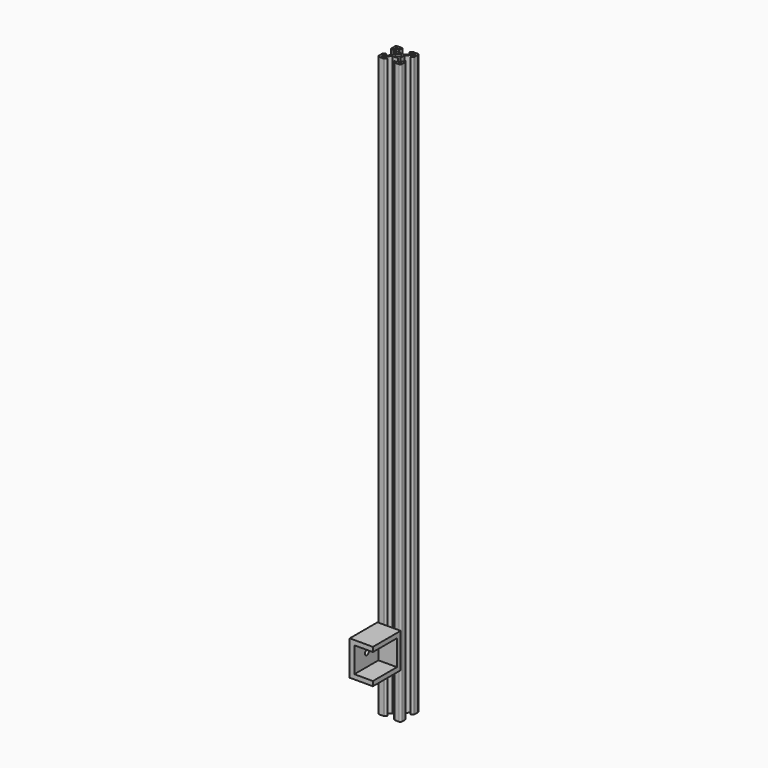
from build123d import *

# Parameters (mm, degrees)
F0_R     = 2.1
F1_DEPTH = 500
F3_W     = 26
F3_H     = 22
F3_R     = 2.15
F4_DEPTH = 20
F7_START = -4
F7_DEPTH = 16


# Not quite as in the source:
# - ends of sketch curves that miss each other by under 0.0002 mm in the source are joined
# - a feature of the source that left no trace in its solid (it failed there, or was rolled back) is left out


with BuildPart() as f1:
    # F0 (on Top) → F1 (new body)
    with BuildSketch(Plane.XY):
        with BuildLine():
            Line((-8.2, 5.5), (-6.56066, 5.5))
            Line((-6.56066, 5.5), (-3.4, 2.33934))
            Line((-3.4, 2.33934), (-3.4, -2.33934))
            Line((-3.4, -2.33934), (-6.56066, -5.5))
            Line((-6.56066, -5.5), (-8.2, -5.5))
            Line((-8.2, -5.5), (-8.2, -2.89))
            Line((-8.2, -2.89), (-8.31, -2.89))
            Line((-8.31, -2.89), (-9.768614, -4.348614))
            ThreePointArc((-9.768614, -4.348614), (-9.9398646954, -4.6049087618), (-10, -4.907229))
            Line((-10, -4.907229), (-10, -8.5))
            ThreePointArc((-10, -8.5), (-9.5606601718, -9.5606601718), (-8.5, -10))
            Line((-8.5, -10), (-4.907229, -10))
            ThreePointArc((-4.907229, -10), (-4.6049087618, -9.9398646954), (-4.3486141429, -9.7686138571))
            Line((-4.3486141429, -9.7686138571), (-2.89, -8.31))
            Line((-2.89, -8.31), (-2.89, -8.2))
            Line((-2.89, -8.2), (-5.5, -8.2))
            Line((-5.5, -8.2), (-5.5, -6.56066))
            Line((-5.5, -6.56066), (-2.33934, -3.4))
            Line((-2.33934, -3.4), (2.33934, -3.4))
            Line((2.33934, -3.4), (5.5, -6.56066))
            Line((5.5, -6.56066), (5.5, -8.2))
            Line((5.5, -8.2), (2.89, -8.2))
            Line((2.89, -8.2), (2.89, -8.31))
            Line((2.89, -8.31), (4.348614, -9.768614))
            ThreePointArc((4.348614, -9.768614), (4.6049087618, -9.9398646954), (4.907229, -10))
            Line((4.907229, -10), (8.5, -10))
            ThreePointArc((8.5, -10), (9.5606601718, -9.5606601718), (10, -8.5))
            Line((10, -8.5), (10, -4.907229))
            ThreePointArc((10, -4.907229), (9.9398646954, -4.6049087618), (9.7686138571, -4.3486141429))
            Line((9.7686138571, -4.3486141429), (8.31, -2.89))
            Line((8.31, -2.89), (8.2, -2.89))
            Line((8.2, -2.89), (8.2, -5.5))
            Line((8.2, -5.5), (6.56066, -5.5))
            Line((6.56066, -5.5), (3.4, -2.33934))
            Line((3.4, -2.33934), (3.4, 2.33934))
            Line((3.4, 2.33934), (6.56066, 5.5))
            Line((6.56066, 5.5), (8.2, 5.5))
            Line((8.2, 5.5), (8.2, 2.89))
            Line((8.2, 2.89), (8.31, 2.89))
            Line((8.31, 2.89), (9.768614, 4.348614))
            ThreePointArc((9.768614, 4.348614), (9.9398646954, 4.6049087618), (10, 4.907229))
            Line((10, 4.907229), (10, 8.5))
            ThreePointArc((10, 8.5), (9.5606601718, 9.5606601718), (8.5, 10))
            Line((8.5, 10), (4.907229, 10))
            ThreePointArc((4.907229, 10), (4.6049087618, 9.9398646954), (4.3486141429, 9.7686138571))
            Line((4.3486141429, 9.7686138571), (2.89, 8.31))
            Line((2.89, 8.31), (2.89, 8.2))
            Line((2.89, 8.2), (5.5, 8.2))
            Line((5.5, 8.2), (5.5, 6.56066))
            Line((5.5, 6.56066), (2.33934, 3.4))
            Line((2.33934, 3.4), (-2.33934, 3.4))
            Line((-2.33934, 3.4), (-5.5, 6.56066))
            Line((-5.5, 6.56066), (-5.5, 8.2))
            Line((-5.5, 8.2), (-2.89, 8.2))
            Line((-2.89, 8.2), (-2.89, 8.31))
            Line((-2.89, 8.31), (-4.348614, 9.768614))
            ThreePointArc((-4.348614, 9.768614), (-4.6049087618, 9.9398646954), (-4.907229, 10))
            Line((-4.907229, 10), (-8.5, 10))
            ThreePointArc((-8.5, 10), (-9.5606601718, 9.5606601718), (-10, 8.5))
            Line((-10, 8.5), (-10, 4.907229))
            ThreePointArc((-10, 4.907229), (-9.9398646954, 4.6049087618), (-9.7686138571, 4.3486141429))
            Line((-9.7686138571, 4.3486141429), (-8.31, 2.89))
            Line((-8.31, 2.89), (-8.2, 2.89))
            Line((-8.2, 2.89), (-8.2, 5.5))
        make_face()
        Polygon((-6.57, -8.2), (-8.2, -8.2), (-8.2, -6.57), (-7.66, -6.57), (-6.57, -7.66), align=None, mode=Mode.SUBTRACT)
        Polygon((6.57, -7.66), (7.66, -6.57), (8.2, -6.57), (8.2, -8.2), (6.57, -8.2), align=None, mode=Mode.SUBTRACT)
        Polygon((-6.57, 7.66), (-7.66, 6.57), (-8.2, 6.57), (-8.2, 8.2), (-6.57, 8.2), align=None, mode=Mode.SUBTRACT)
        Circle(F0_R, mode=Mode.SUBTRACT)
        Polygon((6.57, 8.2), (8.2, 8.2), (8.2, 6.57), (7.66, 6.57), (6.57, 7.66), align=None, mode=Mode.SUBTRACT)
    extrude(amount=F1_DEPTH)


with BuildPart() as f4:
    # F3 (on face) → F4 (new body)
    with BuildSketch(Plane(origin=(-10, 0, 0), x_dir=(0, -1, 0), z_dir=(-1, 0, 0))):
        Polygon((40, 69.6), (10, 69.6), (10, 39.6), (40, 39.6), (40, 43.6), (14, 43.6), (14, 65.6), (40, 65.6), align=None)
        with Locations((27, 54.6)):
            Rectangle(F3_W, F3_H)
        with Locations((26.5, 54.6)):
            Circle(F3_R, mode=Mode.SUBTRACT)
    extrude(amount=-F4_DEPTH)

    # F3 (on face) → F7 (cut)
    with BuildSketch(Plane(origin=(-10, 0, 0), x_dir=(0, -1, 0), z_dir=(-1, 0, 0)).offset(F7_START)):
        with Locations((27, 54.6)):
            Rectangle(F3_W, F3_H)
        with Locations((26.5, 54.6)):
            Circle(F3_R, mode=Mode.SUBTRACT)
    extrude(amount=-F7_DEPTH, mode=Mode.SUBTRACT)


solid = Compound([f1.part, f4.part])
